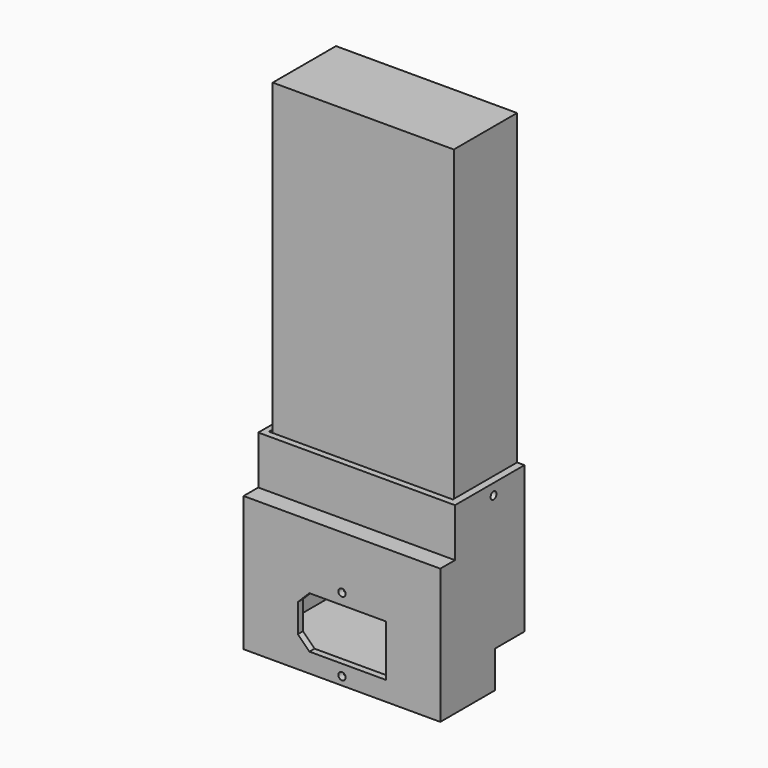
from build123d import *

# Parameters (mm, degrees)
F0_W      = 98.5
F0_H      = 197
F1_DEPTH  = 43
F2_R      = 2
F3_DEPTH  = 10
F4_W      = 43
F4_H      = 29.7
F4_R      = 2
F5_DEPTH  = 4
F7_DEPTH  = 100
F9_DEPTH  = 3
F10_R     = 2.25
F11_DEPTH = 3.5
F12_R     = 2
F13_DEPTH = 3.5
F14_W     = 20
F14_H     = 20
F15_DEPTH = 20


# Not quite as in the source:
# - a feature names something its author has since deleted; it is built from what else it names


with BuildPart() as f1:
    # F0 (on Front) → F1 (new body)
    with BuildSketch(Plane.XZ):
        with Locations((-10.3433534205, 27.6292130947)):
            Rectangle(F0_W, F0_H)
    extrude(amount=F1_DEPTH)

    # F2 (on face) → F3 (cut)
    with BuildSketch(Plane.YZ.offset(38.9066465795)):
        with Locations((-21, -47.1707869053)):
            Circle(F2_R)
    extrude(amount=-F3_DEPTH, mode=Mode.SUBTRACT)


with BuildPart() as f5:
    # F4 (on face) → F5 (new body)
    with BuildSketch(Plane.YZ.offset(38.9066465795)):
        Polygon((-43, -41.1707869053), (-47.2, -41.1707869053), (-47.2, -67.4921646714), (-57.2, -67.4921646714), (-57.2, -140.8707869053), (-47.2, -140.8707869053), (0, -140.8707869053), (0, -70.8707869053), (-43, -70.8707869053), align=None)
        with Locations((-21.5, -56.0207869053)):
            Rectangle(F4_W, F4_H)
        with Locations((-21, -47.1707869053)):
            Circle(F4_R, mode=Mode.SUBTRACT)
    extrude(amount=F5_DEPTH)

    # F6 (on face) → F7 (join)
    with BuildSketch(Plane(origin=(38.9066465795, 0, 0), x_dir=(0, -1, 0), z_dir=(-1, 0, 0))):
        Polygon((43.7, -41.1707869053), (43.7, -44.6707869053), (43.7, -70.9921646714), (53.7, -70.9921646714), (53.7, -137.3707869053), (3.5, -137.3707869053), (3.5, -70.8707869053), (0, -70.8707869053), (0, -140.8707869053), (57.2, -140.8707869053), (57.2, -67.4921646714), (47.2, -67.4921646714), (47.2, -41.1707869053), align=None)
    extrude(amount=F7_DEPTH)

    # F8 (on face) → F9 (join)
    with BuildSketch(Plane(origin=(-61.0933534205, 0, 0), x_dir=(0, -1, 0), z_dir=(-1, 0, 0))):
        Polygon((0, -41.1707869053), (0, -140.8707869053), (57.2, -140.8707869053), (57.2, -67.4921646714), (47.2, -67.4921646714), (47.2, -41.1707869053), (43.7, -41.1707869053), align=None)
    extrude(amount=F9_DEPTH)

    # F10 (on face) → F11 (cut, through all)
    with BuildSketch(Plane(origin=(0, 0, 0), x_dir=(-1, 0, 0), z_dir=(0, 1, 0))):
        with Locations((-14.9066465795, -93.3631800719)):
            Circle(F10_R)
        with BuildLine():
            ThreePointArc((37.8433534205, -93.3631800719), (35.5933534205, -91.1131800719), (33.3433534205, -93.3631800719))
            ThreePointArc((33.3433534205, -93.3631800719), (35.5933534205, -95.6131800719), (37.8433534205, -93.3631800719))
        make_face()
    extrude(amount=-F11_DEPTH, mode=Mode.SUBTRACT)

    # F12 (on face) → F13 (cut, through all)
    with BuildSketch(Plane.XZ.offset(57.2)):
        Polygon((-28.3004602017, -102.3707869053), (-34.5933534205, -108.6636801241), (-34.5933534205, -124.0778936865), (-28.3004602017, -130.3707869053), (13.4066465795, -130.3707869053), (13.4066465795, -102.3707869053), align=None)
        Polygon((-34.0933534205, -108.8707869053), (-28.0933534205, -102.8707869053), (12.9066465795, -102.8707869053), (12.9066465795, -129.8707869053), (-28.0933534205, -129.8707869053), (-34.0933534205, -123.8707869053), align=None, mode=Mode.SUBTRACT)
        Polygon((12.9066465795, -102.8707869053), (-28.0933534205, -102.8707869053), (-34.0933534205, -108.8707869053), (-34.0933534205, -123.8707869053), (-28.0933534205, -129.8707869053), (12.9066465795, -129.8707869053), align=None)
        with Locations((-10.5933534205, -136.3707869053)):
            Circle(F12_R)
        with Locations((-10.5933534205, -96.3707869053)):
            Circle(F12_R)
    extrude(amount=-F13_DEPTH, mode=Mode.SUBTRACT)

    # F14 (on face) → F15 (cut)
    with BuildSketch(Plane(origin=(0, 0, 0), x_dir=(-1, 0, 0), z_dir=(0, 1, 0))):
        with Locations((-32.9066465795, -130.8707869053)):
            Rectangle(F14_W, F14_H)
    extrude(amount=-F15_DEPTH, mode=Mode.SUBTRACT)


solid = Compound([f1.part, f5.part])
